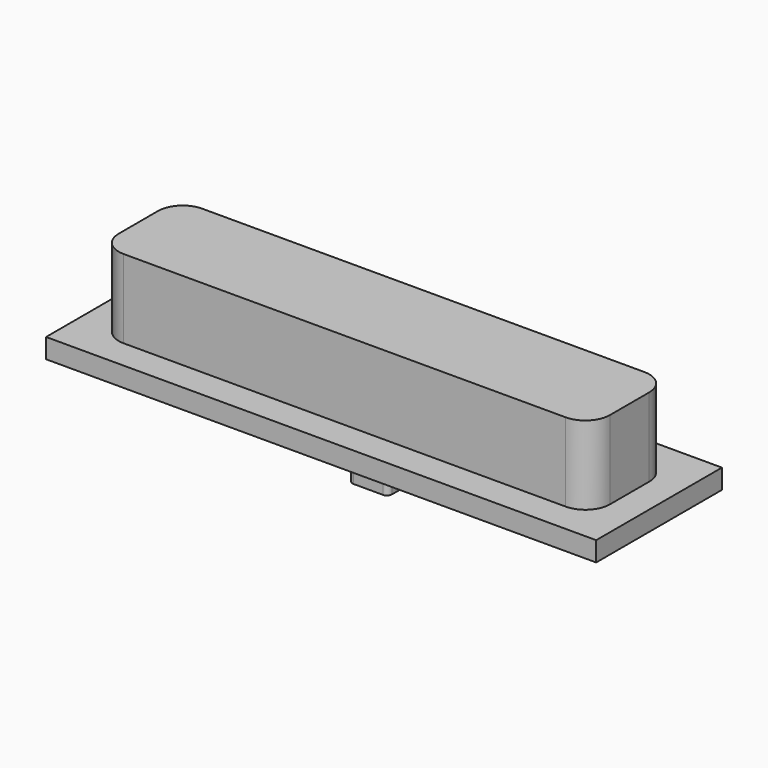
from build123d import *

# Parameters (mm, degrees)
F0_W     = 50
F0_H     = 10
F0_W_2   = 4
F0_H_2   = 4
F0_R     = 1.6
F1_DEPTH = 10
F2_R     = 2.5
F0_W_3   = 56
F0_H_3   = 16
F3_DEPTH = 2
F4_DEPTH = 2
F5_DEPTH = 5
F7_R     = 0.5


# Not quite as in the source:
# - the program builds the solid bodies; features that only make, move or delete a surface that nothing else refers to are left out


with BuildPart() as f1:
    # F0 (on Top) → F1 (new body)
    with BuildSketch(Plane.XY):
        Rectangle(F0_W, F0_H)
        Rectangle(F0_W_2, F0_H_2, mode=Mode.SUBTRACT)
        Rectangle(F0_W_2, F0_H_2)
        Circle(F0_R, mode=Mode.SUBTRACT)
        Circle(F0_R)
    extrude(amount=F1_DEPTH)

    # F2
    f2_edges = [f1.edges().sort_by_distance(p)[0] for p in [
        (-25, -5, 5),
        (-25, 5, 5),
        (25, -5, 5),
        (25, 5, 5),
    ]]
    fillet(f2_edges, radius=F2_R)

    # F0 (on Top) → F3 (join)
    with BuildSketch(Plane.XY):
        Rectangle(F0_W_3, F0_H_3)
        Rectangle(F0_W, F0_H, mode=Mode.SUBTRACT)
    extrude(amount=F3_DEPTH)

    # F0 (on Top) → F4 (join)
    with BuildSketch(Plane.XY):
        Rectangle(F0_W, F0_H)
        Rectangle(F0_W_2, F0_H_2, mode=Mode.SUBTRACT)
    extrude(amount=F4_DEPTH)

    # F0 (on Top) → F5 (join)
    with BuildSketch(Plane.XY):
        Rectangle(F0_W_2, F0_H_2)
        Circle(F0_R, mode=Mode.SUBTRACT)
        Circle(F0_R)
    extrude(amount=-F5_DEPTH)

    # F7
    f7_edges = [f1.edges().sort_by_distance(p)[0] for p in [
        (-2, -2, -2.5),
        (2, -2, -2.5),
        (-2, 2, -2.5),
        (2, 2, -2.5),
    ]]
    fillet(f7_edges, radius=F7_R)


solid = f1.part
